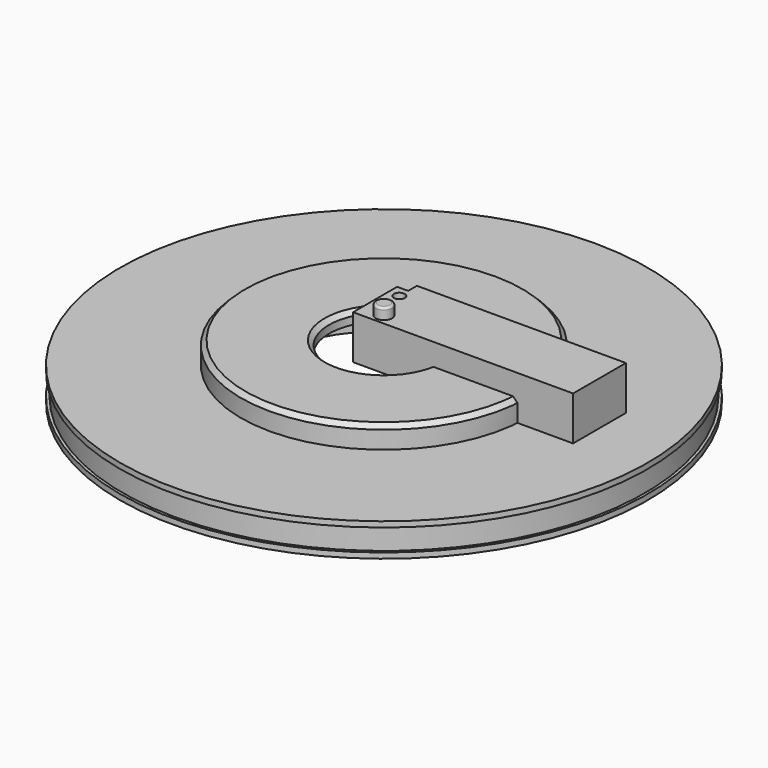
from build123d import *

# Parameters (mm, degrees)
F2_SIZE   = 2.54
F3_W      = 127
F3_H      = 38.1
F4_DEPTH  = 25.4
F5_R      = 4.7625
F6_DEPTH  = 6.35
F7_W      = 6.35
F7_H      = 6.35
F8_DEPTH  = 6.35
F9_R      = 3.175
F10_DEPTH = 6.35
F11_R     = 1.27
F13_W     = 3.175
F13_H     = 12.7


# Not quite as in the source:
# - a feature names something its author has since deleted; it is built from what else it names


with BuildPart() as f1:
    # F0 (on Right) → F1 (revolve)
    with BuildSketch(Plane.YZ):
        Polygon((82.55, 12.7), (31.75, 12.7), (31.75, 5.715), (69.85, 5.715), (69.85, -19.05), (152.4, -19.05), (152.4, 0), (82.55, 0), align=None)
    revolve(axis=Axis((0, 0, 6.35), (0, 0, 1)))

    # F2
    f2_edges = [f1.edges().sort_by_distance(p)[0] for p in [
        (0, -31.75, 12.7),
        (0, -82.55, 12.7),
    ]]
    chamfer(f2_edges, length=F2_SIZE)

    # F13 (on Right) → F14 (revolve, cut)
    with BuildSketch(Plane.YZ):
        with Locations((-152.4, -9.525)):
            Rectangle(F13_W, F13_H)
    revolve(axis=Axis((0, 0, -9.525), (0, 0, -1)), mode=Mode.SUBTRACT)


with BuildPart() as f4:
    # F3 (on Top) → F4 (new body)
    with BuildSketch(Plane.XY):
        with Locations((50.8, 12.7)):
            Rectangle(F3_W, F3_H)
    extrude(amount=F4_DEPTH)

    # F5 (on face) → F6 (join)
    with BuildSketch(Plane.XY.offset(25.4)):
        Circle(F5_R)
    extrude(amount=F6_DEPTH)

    # F7 (on face) → F8 (cut)
    with BuildSketch(Plane.XY.offset(25.4)):
        with Locations((-9.525, 28.575)):
            Rectangle(F7_W, F7_H)
    extrude(amount=-F8_DEPTH, mode=Mode.SUBTRACT)

    # F9 (on face) → F10 (cut)
    with BuildSketch(Plane.XY.offset(25.4)):
        with Locations((-6.35, 19.05)):
            Circle(F9_R)
    extrude(amount=-F10_DEPTH, mode=Mode.SUBTRACT)

    # F11
    f11_edges = [f4.edges().sort_by_distance(p)[0] for p in [
        (-4.7625, 0, 31.75),
    ]]
    fillet(f11_edges, radius=F11_R)


solid = Compound([f1.part, f4.part])
